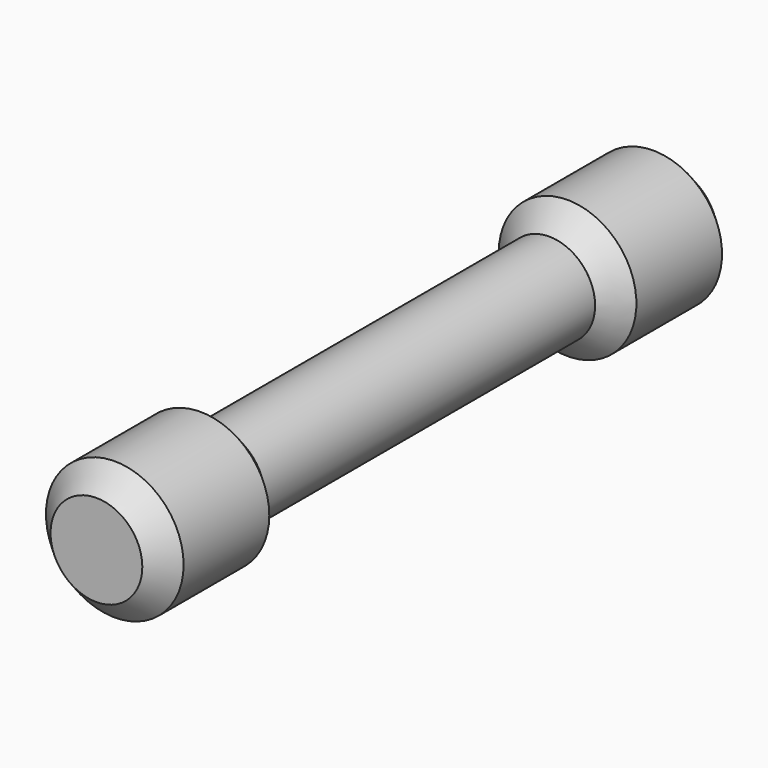
from build123d import *

# Parameters (mm, degrees)
F0_R     = 3
F1_DEPTH = 47
F2_R     = 4.5
F2_R_2   = 3
F3_DEPTH = 10
F4_SIZE  = 1.49999
F5_R     = 4.5
F6_DEPTH = 10
F7_SIZE  = 1.49999


# Not quite as in the source:
# - a fillet or chamfer is up to 0.001 mm smaller than in the source, because OpenCascade refuses the exact size


with BuildPart() as f1:
    # F0 (on Front) → F1 (new body)
    with BuildSketch(Plane.XZ):
        Circle(F0_R)
    extrude(amount=F1_DEPTH)

    # F2 (on face) → F3 (join)
    with BuildSketch(Plane.XZ.offset(47)):
        Circle(F2_R)
        Circle(F2_R_2, mode=Mode.SUBTRACT)
    extrude(amount=-F3_DEPTH)

    # F4 (size 1.5 in the source; OpenCascade refuses exactly that, so slightly less here)
    f4_edges = [f1.edges().sort_by_distance(p)[0] for p in [
        (-4.5, -37, 0),
        (-4.5, -47, 0),
    ]]
    chamfer(f4_edges, length=F4_SIZE)

    # F5 (on face) → F6 (join)
    with BuildSketch(Plane(origin=(0, 0, 0), x_dir=(-1, 0, 0), z_dir=(0, 1, 0))):
        Circle(F5_R)
    extrude(amount=-F6_DEPTH)

    # F7 (size 1.5 in the source; OpenCascade refuses exactly that, so slightly less here)
    f7_edges = [f1.edges().sort_by_distance(p)[0] for p in [
        (4.5, -10, 0),
        (4.5, 0, 0),
    ]]
    chamfer(f7_edges, length=F7_SIZE)


solid = f1.part
